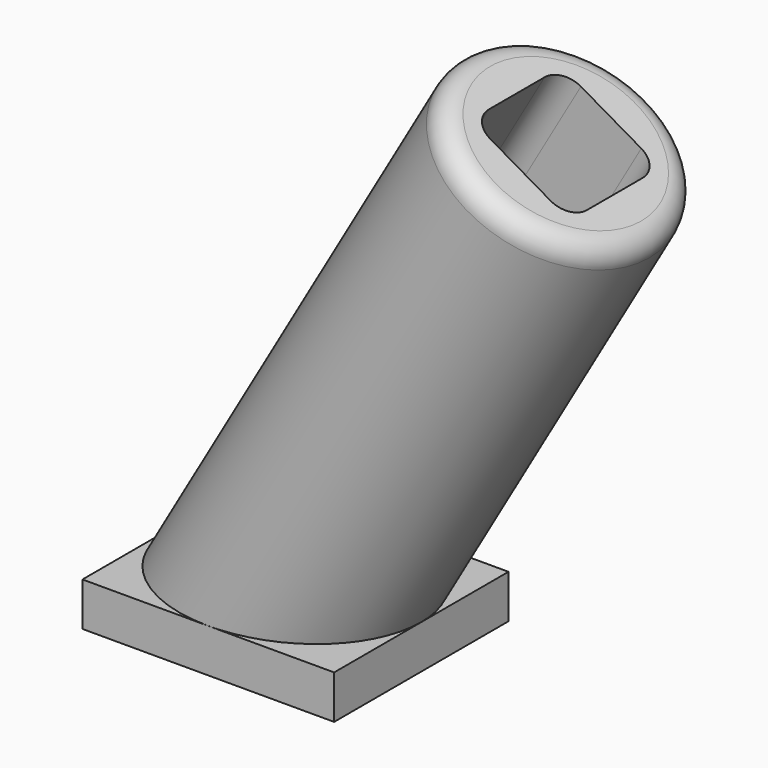
from build123d import *

# Parameters (mm, degrees)
F2_R     = 5
F3_DEPTH = 30
F4_W     = 12.7017059222
F4_H     = 7
F5_DEPTH = 5.5
F6_W     = 11.5470053838
F6_H     = 10
F7_DEPTH = 2
F9_DEPTH = 10
F10_R    = 1


with BuildPart() as f3:
    # F2 (on face) → F3 (new body)
    with BuildSketch(Plane(origin=(0, 0, 0), x_dir=(0.8660254038, 0, -0.5), z_dir=(-0.5, 0, -0.8660254038))):
        with Locations((5, 0)):
            Circle(F2_R)
    extrude(amount=-F3_DEPTH)

    # F4 (on Front) → F5 (cut, symmetric)
    with BuildSketch(Plane.XZ):
        with Locations((6.3508529611, -1.5)):
            Rectangle(F4_W, F4_H)
    extrude(amount=F5_DEPTH, both=True, mode=Mode.SUBTRACT)

    # F6 (on face) → F7 (join)
    with BuildSketch(Plane(origin=(0, 0, 2), x_dir=(1, 0, 0), z_dir=(0, 0, -1))):
        with Locations((6.9282032303, 0)):
            Rectangle(F6_W, F6_H)
    extrude(amount=F7_DEPTH)

    # F8 (on face) → F9 (cut)
    with BuildSketch(Plane(origin=(15, 0, 25.9807621135), x_dir=(0.8660254038, 0, -0.5), z_dir=(0.5, 0, 0.8660254038))):
        with BuildLine():
            Line((6.6, 2.6), (3.4, 2.6))
            ThreePointArc((3.4, 2.6), (2.6928932188, 2.3071067812), (2.4, 1.6))
            Line((2.4, 1.6), (2.4, -1.6))
            ThreePointArc((2.4, -1.6), (2.6928932188, -2.3071067812), (3.4, -2.6))
            Line((3.4, -2.6), (6.6, -2.6))
            ThreePointArc((6.6, -2.6), (7.3071067812, -2.3071067812), (7.6, -1.6))
            Line((7.6, -1.6), (7.6, 1.6))
            ThreePointArc((7.6, 1.6), (7.3071067812, 2.3071067812), (6.6, 2.6))
        make_face()
    extrude(amount=-F9_DEPTH, mode=Mode.SUBTRACT)

    # F10
    f10_edges = [f3.edges().sort_by_distance(p)[0] for p in [
        (15, 0, 25.980762),
    ]]
    fillet(f10_edges, radius=F10_R)


solid = f3.part
